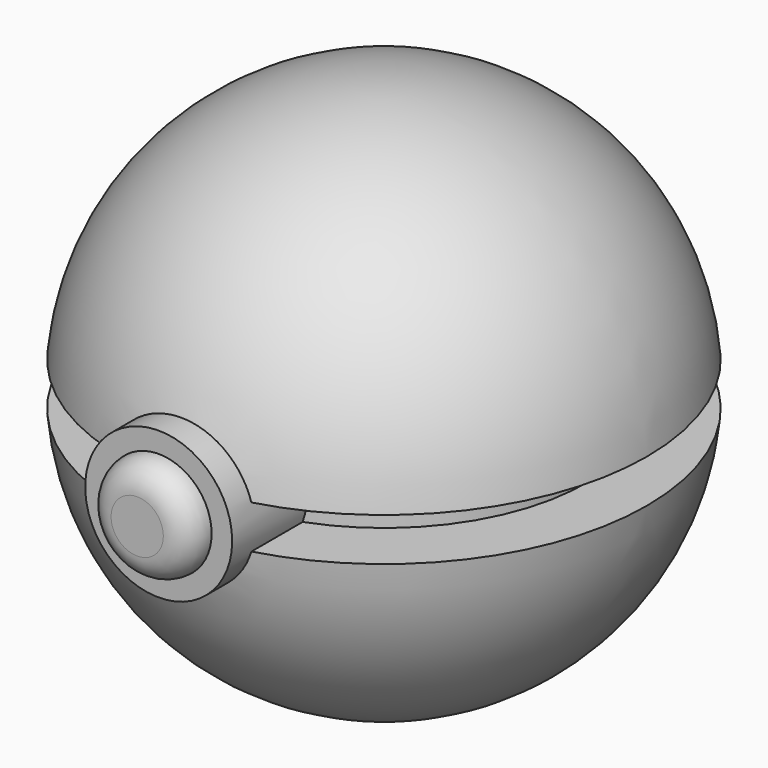
from build123d import *

# Parameters (mm, degrees)
F2_R     = 13.922185385
F3_DEPTH = 53.34
F4_R     = 10.0272817178
F5_DEPTH = 5.08
F6_R     = 5.07999


# Not quite as in the source:
# - a fillet or chamfer is up to 0.001 mm smaller than in the source, because OpenCascade refuses the exact size


with BuildPart() as f1:
    # F0 (on Front) → F1 (revolve)
    with BuildSketch(Plane.XZ):
        with BuildLine():
            Line((0, 0), (0, -50))
            ThreePointArc((0, -50), (33.8768500277, -36.7744344919), (49.8320800855, -4.0943612879))
            Line((49.8320800855, -4.0943612879), (38.2781662047, -4.0943612879))
            Line((38.2781662047, -4.0943612879), (38.2781662047, 0))
            Line((38.2781662047, 0), (38.2781662047, 4.0943612879))
            Line((38.2781662047, 4.0943612879), (49.8320800855, 4.0943612879))
            ThreePointArc((49.8320800855, 4.0943612879), (33.8768500277, 36.7744344919), (0, 50))
            Line((0, 50), (0, 0))
        make_face()
    revolve(axis=Axis((0, 0, 25), (0, 0, 1)))

    # F2 (on Front) → F3 (join)
    with BuildSketch(Plane.XZ):
        Circle(F2_R)
    extrude(amount=F3_DEPTH)

    # F4 (on face) → F5 (join)
    with BuildSketch(Plane.XZ.offset(53.34)):
        Circle(F4_R)
    extrude(amount=F5_DEPTH)

    # F6 (radius 5.08 in the source; OpenCascade refuses exactly that, so slightly less here)
    f6_edges = [f1.edges().sort_by_distance(p)[0] for p in [
        (-10.027282, -58.42, 0),
    ]]
    fillet(f6_edges, radius=F6_R)


solid = f1.part
